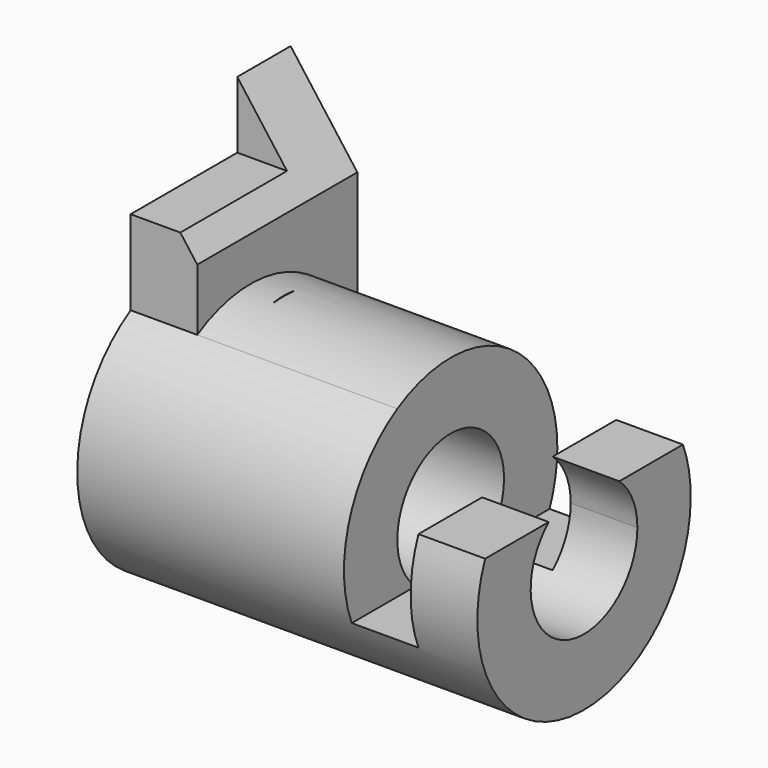
from build123d import *

# Parameters (mm, degrees)
F0_R          = 12.7
F1_DEPTH      = 76.2
F3_DEPTH      = 25.401
F3_DEPTH_BACK = 25.4
F5_DEPTH      = 63.5
F7_DEPTH      = 25.4
F7_DEPTH_BACK = 25.4


with BuildPart() as f1:
    # F0 (on Right) → F1 (new body)
    with BuildSketch(Plane.YZ):
        with BuildLine():
            ThreePointArc((-12.7, 21.997045), (-12.7, -21.997045), (25.4, 0))
            ThreePointArc((25.4, 0), (12.7, 21.997045), (-12.7, 21.997045))
        make_face()
        Circle(F0_R, mode=Mode.SUBTRACT)
        with BuildLine():
            ThreePointArc((-12.7, 21.997045), (12.7, 21.997045), (25.4, 0))
            Line((25.4, 0), (25.4, 50.8))
            Line((25.4, 50.8), (12.7, 50.8))
            Line((12.7, 50.8), (12.7, 38.1))
            Line((12.7, 38.1), (-12.7, 38.1))
            Line((-12.7, 38.1), (-12.7, 21.997045))
        make_face()
    extrude(amount=F1_DEPTH)

    # F2 (on Front) → F3 (cut, two sides)
    with BuildSketch(Plane.XZ) as f3_sk:
        Polygon((63.5, 25.4), (50.8, 25.4), (50.8, -9.525), (63.5, -9.525), (63.5, 9.525), (76.2, 9.525), (76.2, 25.4), align=None)
    extrude(amount=-F3_DEPTH, mode=Mode.SUBTRACT)
    extrude(f3_sk.sketch, amount=F3_DEPTH_BACK, mode=Mode.SUBTRACT)

    # F4 (on face) → F5 (cut)
    with BuildSketch(Plane.YZ.offset(76.2)):
        with BuildLine():
            ThreePointArc((-12.7, 21.997045), (12.7, 21.997045), (25.4, 0))
            Line((25.4, 0), (25.4, 25.4))
            Line((25.4, 25.4), (25.4, 50.8))
            Line((25.4, 50.8), (12.7, 50.8))
            Line((12.7, 50.8), (12.7, 38.1))
            Line((12.7, 38.1), (-12.7, 38.1))
            Line((-12.7, 38.1), (-12.7, 21.997045))
        make_face()
    extrude(amount=-F5_DEPTH, mode=Mode.SUBTRACT)

    # F6 (on Front) → F7 (cut, two sides)
    with BuildSketch(Plane.XZ) as f7_sk:
        Polygon((0, 50.8), (19.05, 25.25617), (19.05, 50.8), align=None)
    extrude(amount=-F7_DEPTH, mode=Mode.SUBTRACT)
    extrude(f7_sk.sketch, amount=F7_DEPTH_BACK, mode=Mode.SUBTRACT)


solid = f1.part
